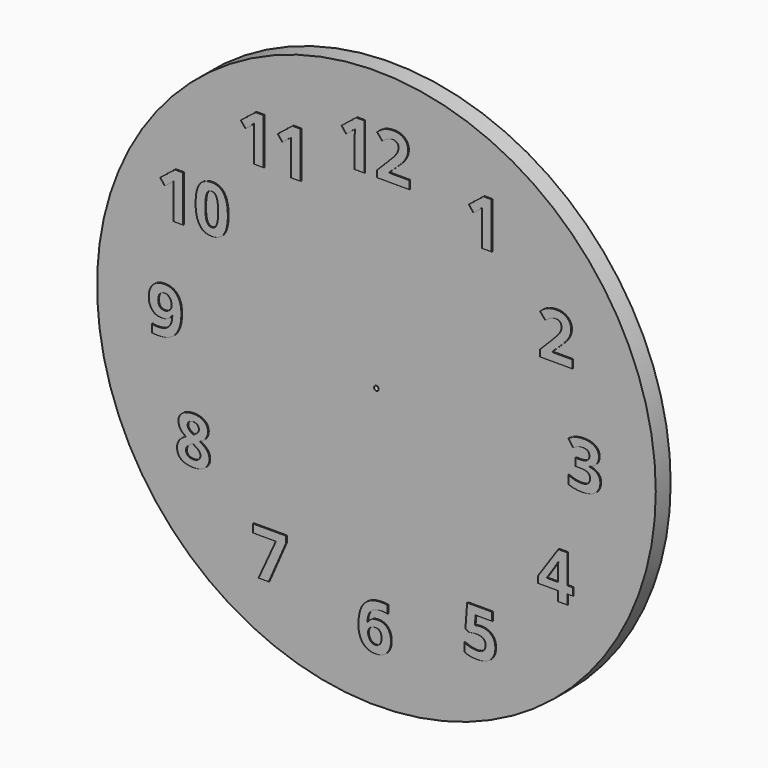
from build123d import *

# Parameters (mm, degrees)
F0_R         = 76.2
F0_R_2       = 0.635
F1_DEPTH     = 5.08
F3_TEXT_SIZE = 17.6388888889
F4_DEPTH     = 0.254


# Not quite as in the source:
# - Text() gives the source's letters only with a copy of the font that has no kerning and outlines rounded to 1/6400 em; it was checked with that copy


with BuildPart() as f1:
    # F0 (on Front) → F1 (new body)
    with BuildSketch(Plane.XZ):
        Circle(F0_R)
        Circle(F0_R_2, mode=Mode.SUBTRACT)
    extrude(amount=F1_DEPTH)

    # F3 (on face) → F4 (join)
    with BuildSketch(Plane.XZ.offset(5.08)):
        with Locations((24.3595811632, 43.1433518263)):
            Text('1', F3_TEXT_SIZE, font='Open Sans', font_style=FontStyle.BOLD, text_align=(TextAlign.LEFT, TextAlign.BOTTOM))
        with Locations((44.1672342048, 22.225)):
            Text('2', F3_TEXT_SIZE, font='Open Sans', font_style=FontStyle.BOLD, text_align=(TextAlign.LEFT, TextAlign.BOTTOM))
        with Locations((51.884516059, -6.35)):
            Text('3', F3_TEXT_SIZE, font='Open Sans', font_style=FontStyle.BOLD, text_align=(TextAlign.LEFT, TextAlign.BOTTOM))
        with Locations((44.0252962707, -34.925)):
            Text('4', F3_TEXT_SIZE, font='Open Sans', font_style=FontStyle.BOLD, text_align=(TextAlign.LEFT, TextAlign.BOTTOM))
        with Locations((23.3646375868, -55.8433518263)):
            Text('5', F3_TEXT_SIZE, font='Open Sans', font_style=FontStyle.BOLD, text_align=(TextAlign.LEFT, TextAlign.BOTTOM))
        with Locations((-5.3261176215, -63.5)):
            Text('6', F3_TEXT_SIZE, font='Open Sans', font_style=FontStyle.BOLD, text_align=(TextAlign.LEFT, TextAlign.BOTTOM))
        with Locations((-33.9011176215, -55.8433518263)):
            Text('7', F3_TEXT_SIZE, font='Open Sans', font_style=FontStyle.BOLD, text_align=(TextAlign.LEFT, TextAlign.BOTTOM))
        with Locations((-54.7932867221, -34.925)):
            Text('8', F3_TEXT_SIZE, font='Open Sans', font_style=FontStyle.BOLD, text_align=(TextAlign.LEFT, TextAlign.BOTTOM))
        with Locations((-62.4499348958, -6.35)):
            Text('9', F3_TEXT_SIZE, font='Open Sans', font_style=FontStyle.BOLD, text_align=(TextAlign.LEFT, TextAlign.BOTTOM))
        with Locations((-59.8189920173, 22.225)):
            Text('10', F3_TEXT_SIZE, font='Open Sans', font_style=FontStyle.BOLD, text_align=(TextAlign.LEFT, TextAlign.BOTTOM))
        with Locations((-37.8243923611, 43.1433518263)):
            Text('11', F3_TEXT_SIZE, font='Open Sans', font_style=FontStyle.BOLD, text_align=(TextAlign.LEFT, TextAlign.BOTTOM))
        with Locations((-10.3600911458, 50.8)):
            Text('12', F3_TEXT_SIZE, font='Open Sans', font_style=FontStyle.BOLD, text_align=(TextAlign.LEFT, TextAlign.BOTTOM))
    extrude(amount=F4_DEPTH)


solid = f1.part
